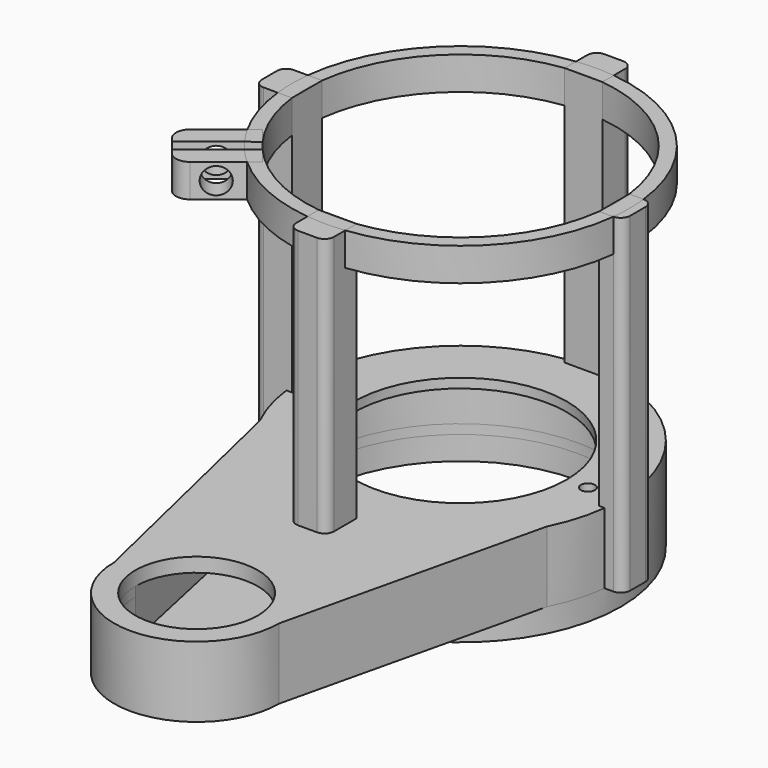
from build123d import *

# Parameters (mm, degrees)
F1_DEPTH  = 15
F3_START  = -2
F2_R      = 31
F3_DEPTH  = 19.9
F5_START  = -3
F5_DEPTH  = 10
F6_R      = 22.5
F6_R_2    = 13
F7_DEPTH  = 5
F10_R     = 34
F10_R_2   = 31
F11_DEPTH = 5
F12_R     = 1.5
F13_DEPTH = 5
F15_DEPTH = 70
F16_R     = 35.825
F16_R_2   = 32.825
F17_DEPTH = 7
F19_DEPTH = 9.7
F21_DEPTH = 7
F22_R     = 2.75
F23_DEPTH = 14.84


# Not quite as in the source:
# - the program builds the solid bodies; features that only make, move or delete a surface that nothing else refers to are left out


with BuildPart() as f1:
    # F0 (on Top) → F1 (new body)
    with BuildSketch(Plane.XY):
        with BuildLine():
            Line((30.4207066557, -15.1848808546), (34, 0))
            ThreePointArc((34, 0), (0, 34), (-34, 0))
            Line((-34, 0), (-30.4207066557, -15.1848808546))
            ThreePointArc((-30.4207066557, -15.1848808546), (0, -34), (30.4207066557, -15.1848808546))
        make_face()
        with BuildLine():
            ThreePointArc((30.4207066557, -15.1848808546), (33.0930810465, -7.8005119609), (34, 0))
            Line((34, 0), (30.4207066557, -15.1848808546))
        make_face()
        with BuildLine():
            Line((-30.4207066557, -15.1848808546), (-34, 0))
            ThreePointArc((-34, 0), (-33.0930810465, -7.8005119609), (-30.4207066557, -15.1848808546))
        make_face()
        with BuildLine():
            Line((17.5, -70), (30.4207066557, -15.1848808546))
            ThreePointArc((30.4207066557, -15.1848808546), (0, -34), (-30.4207066557, -15.1848808546))
            Line((-30.4207066557, -15.1848808546), (-17.5, -70))
            ThreePointArc((-17.5, -70), (0, -52.5), (17.5, -70))
        make_face()
        with BuildLine():
            ThreePointArc((-17.5, -70), (0, -87.5), (17.5, -70))
            ThreePointArc((17.5, -70), (0, -52.5), (-17.5, -70))
        make_face()
    extrude(amount=F1_DEPTH)

    # F2 (on face) → F3 (cut)
    with BuildSketch(Plane.XY.offset(15).offset(F3_START)):
        Circle(F2_R)
    extrude(amount=-F3_DEPTH, mode=Mode.SUBTRACT)

    # F4 (on face) → F5 (cut)
    with BuildSketch(Plane.XY.offset(15).offset(F5_START)):
        with BuildLine():
            ThreePointArc((-13, -70), (0, -83), (13, -70))
            ThreePointArc((13, -70), (0, -57), (-13, -70))
        make_face()
        with BuildLine():
            ThreePointArc((-13, -70), (0, -57), (13, -70))
            Line((13, -70), (23.8560199829, -19.7962196031))
            ThreePointArc((23.8560199829, -19.7962196031), (0, -31), (-23.8560199829, -19.7962196031))
            Line((-23.8560199829, -19.7962196031), (-13, -70))
        make_face()
        with BuildLine():
            ThreePointArc((-23.8560199829, -19.7962196031), (0, -31), (23.8560199829, -19.7962196031))
            ThreePointArc((23.8560199829, -19.7962196031), (29.1593605852, -10.5229126322), (31, 0))
            ThreePointArc((31, 0), (-10.5229126322, 29.1593605852), (-23.8560199829, -19.7962196031))
        make_face()
    extrude(amount=-F5_DEPTH, mode=Mode.SUBTRACT)

    # F6 (on face) → F7 (cut)
    with BuildSketch(Plane.XY.offset(15)):
        Circle(F6_R)
        with Locations((0, -70)):
            Circle(F6_R_2)
    extrude(amount=-F7_DEPTH, mode=Mode.SUBTRACT)

    # F10 (on face) → F11 (join)
    with BuildSketch(Plane(origin=(0, 0, 0), x_dir=(1, 0, 0), z_dir=(0, 0, -1))):
        Circle(F10_R)
        Circle(F10_R_2, mode=Mode.SUBTRACT)
    extrude(amount=F11_DEPTH)

    # F12 (on face) → F13 (cut)
    with BuildSketch(Plane.XY.offset(15)):
        with Locations((-27, 0)):
            Circle(F12_R)
        with Locations((27, 0)):
            Circle(F12_R)
    extrude(amount=-F13_DEPTH, mode=Mode.SUBTRACT)

    # F14 (on Top) → F15 (join)
    with BuildSketch(Plane.XY):
        with BuildLine():
            ThreePointArc((-40.580371775, -2), (-39.9945853374, -3.4142135624), (-38.580371775, -4))
            Line((-38.580371775, -4), (-32.580371775, -4))
            Line((-32.580371775, -4), (-32.580371775, 4))
            Line((-32.580371775, 4), (-38.580371775, 4))
            ThreePointArc((-38.580371775, 4), (-39.9945853374, 3.4142135624), (-40.580371775, 2))
            Line((-40.580371775, 2), (-40.580371775, -2))
        make_face()
        with BuildLine():
            Line((-4, 38.580371775), (-4, 32.580371775))
            Line((-4, 32.580371775), (4, 32.580371775))
            Line((4, 32.580371775), (4, 38.580371775))
            ThreePointArc((4, 38.580371775), (3.4142135624, 39.9945853374), (2, 40.580371775))
            Line((2, 40.580371775), (-2, 40.580371775))
            ThreePointArc((-2, 40.580371775), (-3.4142135624, 39.9945853374), (-4, 38.580371775))
        make_face()
        with BuildLine():
            Line((32.580371775, 4), (32.580371775, -4))
            Line((32.580371775, -4), (35.580371775, -4))
            ThreePointArc((35.580371775, -4), (36.9945853374, -3.4142135624), (37.580371775, -2))
            Line((37.580371775, -2), (37.580371775, 2))
            ThreePointArc((37.580371775, 2), (36.9945853374, 3.4142135624), (35.580371775, 4))
            Line((35.580371775, 4), (32.580371775, 4))
        make_face()
        with BuildLine():
            Line((4, -32.580371775), (-4, -32.580371775))
            Line((-4, -32.580371775), (-4, -38.580371775))
            ThreePointArc((-4, -38.580371775), (-3.4142135624, -39.9945853374), (-2, -40.580371775))
            Line((-2, -40.580371775), (2, -40.580371775))
            ThreePointArc((2, -40.580371775), (3.4142135624, -39.9945853374), (4, -38.580371775))
            Line((4, -38.580371775), (4, -32.580371775))
        make_face()
    extrude(amount=F15_DEPTH)

    # F16 (on face) → F17 (join)
    with BuildSketch(Plane.XY.offset(70)):
        Circle(F16_R)
        Circle(F16_R_2, mode=Mode.SUBTRACT)
    extrude(amount=-F17_DEPTH)

    # F18 (on face) → F19 (cut)
    with BuildSketch(Plane.XY.offset(70)):
        Polygon((-23.3274125101, -16.7493631263), (-31.6316734562, -23.3615097559), (-29.853291891, -25.5949969131), (-21.5490309449, -18.9828502835), align=None)
    extrude(amount=-F19_DEPTH, mode=Mode.SUBTRACT)

    # F20 (on face) → F21 (join)
    with BuildSketch(Plane.XY.offset(70)):
        with BuildLine():
            Line((-38.2785545197, -28.6539918331), (-26.5440042016, -19.3105273347))
            Line((-26.5440042016, -19.3105273347), (-29.2896663374, -15.8622228547))
            Line((-29.2896663374, -15.8622228547), (-38.6773065919, -23.3369944533))
            ThreePointArc((-38.6773065919, -23.3369944533), (-39.7894951343, -25.3457539175), (-39.1555237558, -27.5525974166))
            Line((-39.1555237558, -27.5525974166), (-38.2785545197, -28.6539918331))
        make_face()
        with BuildLine():
            Line((-22.0199605007, -24.9923189719), (-24.7656226365, -21.5440144919))
            Line((-24.7656226365, -21.5440144919), (-36.5001729546, -30.8874789902))
            Line((-36.5001729546, -30.8874789902), (-35.6232037185, -31.9888734067))
            ThreePointArc((-35.6232037185, -31.9888734067), (-33.6144442544, -33.1010619491), (-31.4076007552, -32.4670905706))
            Line((-31.4076007552, -32.4670905706), (-22.0199605007, -24.9923189719))
        make_face()
    extrude(amount=-F21_DEPTH)

    # F22 (on face) → F23 (cut)
    with BuildSketch(Plane(origin=(3.6348529183, -4.5650480586, 0), x_dir=(0.7823033545, 0.6228976332, 0), z_dir=(0.6228976332, -0.7823033545, 0))):
        with Locations((-40.469146122, 66.5)):
            Circle(F22_R)
    extrude(amount=-F23_DEPTH, mode=Mode.SUBTRACT)


solid = f1.part
